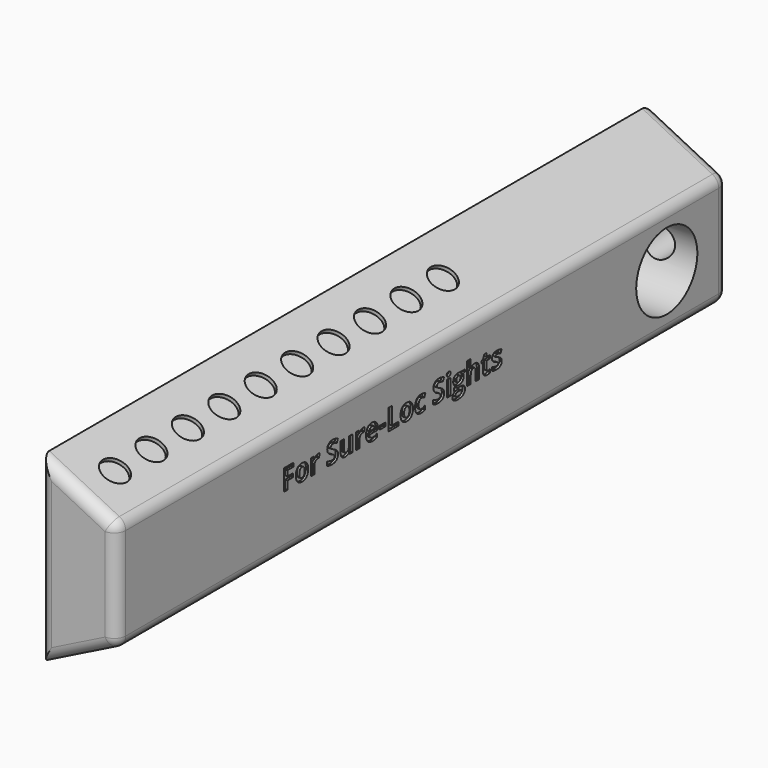
from build123d import *

# Parameters (mm, degrees)
F1_DEPTH      = 5
F3_DEPTH      = 100.001
F5_D          = 4.2
F5_DEPTH      = 10
F5_TIP        = 1.2618073
F6_R          = 5
F7_DEPTH      = 10.001
F8_R          = 1.75
F9_DEPTH      = 0.5
F10_R         = 1.75
F11_DEPTH     = 0.5
F12_TEXT_SIZE = 3.8310626729
F13_DEPTH     = 0.3
F14_R         = 1.5


# Not quite as in the source:
# - Text() gives the source's letters only with a copy of the font that has no kerning and outlines rounded to 1/6400 em; it was checked with that copy


with BuildPart() as f1:
    # F0 (on Right) → F1 (new body, symmetric)
    with BuildSketch(Plane.YZ):
        Polygon((50, 7), (50, 12), (-50, 12), (-50, -7), (-50, -12), (50, -12), align=None)
    extrude(amount=F1_DEPTH, both=True)

    # F2 (on face) → F3 (cut, through all)
    with BuildSketch(Plane(origin=(0, 50, 0), x_dir=(-1, 0, 0), z_dir=(0, 1, 0))):
        Polygon((-5, 12), (-5, 7), (5, 12), align=None)
        Polygon((5, -12), (-5, -7), (-5, -12), align=None)
    extrude(amount=-F3_DEPTH, mode=Mode.SUBTRACT)

    # F5
    with Locations(Plane(origin=(0, 50, 0), x_dir=(-1, 0, 0), z_dir=(0, 1, 0))):
        with Locations((0, 0)):
            Hole(F5_D / 2, depth=F5_DEPTH)
            with Locations((0, 0, -(F5_DEPTH + F5_TIP / 2))):  # 118° drill point
                Cone(0, F5_D / 2, F5_TIP, mode=Mode.SUBTRACT)

    # F6 (on face) → F7 (cut, through all)
    with BuildSketch(Plane(origin=(-5, 0, 0), x_dir=(0, -1, 0), z_dir=(-1, 0, 0))):
        with Locations((-40, 0)):
            Circle(F6_R)
    extrude(amount=-F7_DEPTH, mode=Mode.SUBTRACT)

    # F8 (on face) → F9 (cut)
    with BuildSketch(Plane(origin=(3.8, 0, 7.6), x_dir=(0.894427191, 0, -0.4472135955), z_dir=(0.4472135955, 0, 0.894427191))):
        with Locations((-4.2485291572, -44)):
            Circle(F8_R)
        with Locations((-4.2855792171, -38.0001143933)):
            Circle(F8_R)
        with Locations((-4.322629277, -32.0002287867)):
            Circle(F8_R)
        with Locations((-4.3596793368, -26.00034318)):
            Circle(F8_R)
        with Locations((-4.3967293967, -20.0004575733)):
            Circle(F8_R)
        with Locations((-4.4337794566, -14.0005719667)):
            Circle(F8_R)
        with Locations((-4.4708295164, -8.00068636)):
            Circle(F8_R)
        with Locations((-4.5078795763, -2.0008007533)):
            Circle(F8_R)
        with Locations((-4.5449296361, 3.9990848533)):
            Circle(F8_R)
        with Locations((-4.581979696, 9.99897046)):
            Circle(F8_R)
    extrude(amount=-F9_DEPTH, mode=Mode.SUBTRACT)

    # F10 (on face) → F11 (cut)
    with BuildSketch(Plane(origin=(3.8, 0, -7.6), x_dir=(0.894427191, 0, 0.4472135955), z_dir=(0.4472135955, 0, -0.894427191))):
        with Locations((-4.2485291572, 44)):
            Circle(F10_R)
        with Locations((-4.2378677275, 38.0000094722)):
            Circle(F10_R)
        with Locations((-4.2272062978, 32.0000189444)):
            Circle(F10_R)
        with Locations((-4.2165448681, 26.0000284165)):
            Circle(F10_R)
        with Locations((-4.2058834383, 20.0000378887)):
            Circle(F10_R)
        with Locations((-4.1952220086, 14.0000473609)):
            Circle(F10_R)
        with Locations((-4.1845605789, 8.0000568331)):
            Circle(F10_R)
        with Locations((-4.1738991491, 2.0000663053)):
            Circle(F10_R)
        with Locations((-4.1632377194, -3.9999242226)):
            Circle(F10_R)
        with Locations((-4.1525762897, -9.9999147504)):
            Circle(F10_R)
    extrude(amount=-F11_DEPTH, mode=Mode.SUBTRACT)

    # F12 (on face) → F13 (cut)
    with BuildSketch(Plane.YZ.offset(5)):
        with Locations((-22.9530745358, 0)):
            Text('For Sure-Loc Sights', F12_TEXT_SIZE, font='Open Sans', font_style=FontStyle.BOLD, text_align=(TextAlign.LEFT, TextAlign.BOTTOM))
    extrude(amount=-F13_DEPTH, mode=Mode.SUBTRACT)

    # F14
    f14_edges = [f1.edges().sort_by_distance(p)[0] for p in [
        (5, 0, 7),
        (5, 0, -7),
        (0, -50, 9.5),
        (5, -50, 0),
        (0, -50, -9.5),
        (0, 50, -9.5),
        (0, 50, 9.5),
        (5, 50, 0),
        (-5, 50, 0),
        (-5, -50, 0),
    ]]
    fillet(f14_edges, radius=F14_R)


solid = f1.part
